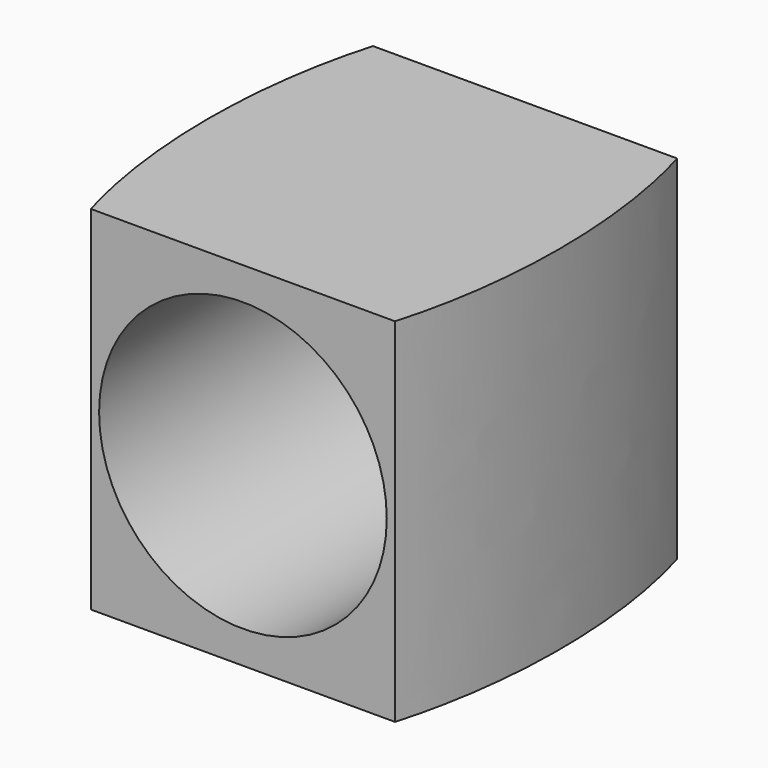
from build123d import *

# Parameters (mm, degrees)
F0_W          = 21.7
F0_H          = 21.7
F0_R          = 8.85
F1_DEPTH      = 10.85
F1_DEPTH_BACK = 10.85
F3_DEPTH      = 25


with BuildPart() as f1:
    # F0 (on Front) → F1 (new body, two sides)
    with BuildSketch(Plane.XZ) as f1_sk:
        Rectangle(F0_W, F0_H)
        Circle(F0_R, mode=Mode.SUBTRACT)
    extrude(amount=F1_DEPTH)
    extrude(f1_sk.sketch, amount=-F1_DEPTH_BACK)

    # F2 (on face) → F3 (cut)
    with BuildSketch(Plane.XY.offset(10.85)):
        with BuildLine():
            add(Edge.make_bspline(
                [(7.9357599601, -14.6792419255), (8.7533080621, -12.9220378395), (9.3575897376, -10.85)],
                knots=[0.8228915355, 0.8228915355, 0.8228915355, 1.0440868221, 1.0440868221, 1.0440868221], degree=2, weights=[1, 0.9938903122, 1]))
            Line((7.9357599601, -14.6792419255), (17.9156405647, -14.6792419255))
            Line((17.9156405647, -14.6792419255), (17.9156405647, 12.7848008303))
            Line((17.9156405647, 12.7848008303), (8.7213948385, 12.7848008303))
            add(Edge.make_bspline(
                [(9.3575897376, 10.85), (9.0655324995, 11.8514429913), (8.7213948385, 12.7848008303)],
                knots=[2.0975058315, 2.0975058315, 2.0975058315, 2.2047475395, 2.2047475395, 2.2047475395], degree=2, weights=[1, 0.9985627464, 1]))
            Line((9.3575897376, 10.85), (10.85, 10.85))
            Line((10.85, 10.85), (10.85, -10.85))
            Line((10.85, -10.85), (9.3575897376, -10.85))
        make_face()
        with BuildLine():
            Line((-17.9156405647, -14.6792419255), (-7.9357599601, -14.6792419255))
            add(Edge.make_bspline(
                [(-9.3575897376, -10.85), (-8.7533080621, -12.9220378395), (-7.9357599601, -14.6792419255)],
                knots=[5.2390984851, 5.2390984851, 5.2390984851, 5.4602937717, 5.4602937717, 5.4602937717], degree=2, weights=[1, 0.9938903122, 1]))
            Line((-9.3575897376, -10.85), (-10.85, -10.85))
            Line((-10.85, -10.85), (-10.85, 10.85))
            Line((-10.85, 10.85), (-9.3575897376, 10.85))
            add(Edge.make_bspline(
                [(-8.7213948385, 12.7848008303), (-9.0655324995, 11.8514429913), (-9.3575897376, 10.85)],
                knots=[4.0784377676, 4.0784377676, 4.0784377676, 4.1856794756, 4.1856794756, 4.1856794756], degree=2, weights=[1, 0.9985627464, 1]))
            Line((-8.7213948385, 12.7848008303), (-17.9156405647, 12.7848008303))
            Line((-17.9156405647, 12.7848008303), (-17.9156405647, -14.6792419255))
        make_face()
        with BuildLine():
            add(Edge.make_bspline(
                [(9.3575897376, -10.85), (12.5218447792, 0), (9.3575897376, 10.85)],
                knots=[1.0440868221, 1.0440868221, 1.0440868221, 2.0975058315, 2.0975058315, 2.0975058315], degree=2, weights=[1, 0.8644658516, 1]))
            Line((9.3575897376, -10.85), (10.85, -10.85))
            Line((10.85, -10.85), (10.85, 10.85))
            Line((10.85, 10.85), (9.3575897376, 10.85))
        make_face()
        with BuildLine():
            Line((-10.85, -10.85), (-9.3575897376, -10.85))
            add(Edge.make_bspline(
                [(-9.3575897376, 10.85), (-12.5218447792, 0), (-9.3575897376, -10.85)],
                knots=[4.1856794756, 4.1856794756, 4.1856794756, 5.2390984851, 5.2390984851, 5.2390984851], degree=2, weights=[1, 0.8644658516, 1]))
            Line((-9.3575897376, 10.85), (-10.85, 10.85))
            Line((-10.85, 10.85), (-10.85, -10.85))
        make_face()
    extrude(amount=-F3_DEPTH, mode=Mode.SUBTRACT)


solid = f1.part
